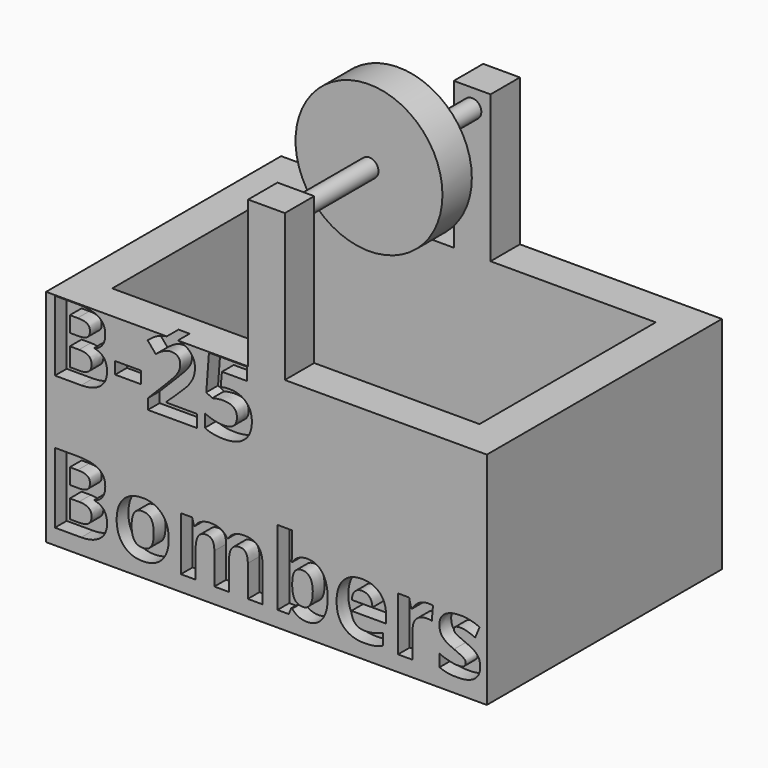
from build123d import *

# Parameters (mm, degrees)
F0_W          = 152.4
F0_H          = 76.2
F1_DEPTH      = 101.6
F2_W          = 127
F2_H          = 76.2
F3_DEPTH      = 63.5
F4_W          = 76.2
F4_H          = 25.4
F5_DEPTH      = 12.7
F6_W          = 12.7
F6_H          = 12.7
F7_DEPTH      = 50.8
F8_W          = 12.7
F8_H          = 12.7
F9_DEPTH      = 50.8
F10_R         = 3.175
F11_DEPTH     = 101.6
F13_R         = 25.4
F14_DEPTH     = 6.35
F15_R         = 6.35
F16_DEPTH     = 76.2
F17_TEXT_SIZE = 34.039085564
F18_DEPTH     = 5.08


# Not quite as in the source:
# - Text() gives the source's letters only with a copy of the font that has no kerning and outlines rounded to 1/6400 em; it was checked with that copy


with BuildPart() as f1:
    # F0 (on Front) → F1 (new body)
    with BuildSketch(Plane.XZ):
        with Locations((76.2, 38.1)):
            Rectangle(F0_W, F0_H)
    extrude(amount=-F1_DEPTH)

    # F2 (on face) → F3 (cut)
    with BuildSketch(Plane.XY.offset(76.2)):
        with Locations((76.2, 50.8)):
            Rectangle(F2_W, F2_H)
    extrude(amount=-F3_DEPTH, mode=Mode.SUBTRACT)

    # F4 (on face) → F5 (cut)
    with BuildSketch(Plane.XY.offset(12.7)):
        with Locations((76.2, 50.8)):
            Rectangle(F4_W, F4_H)
    extrude(amount=-F5_DEPTH, mode=Mode.SUBTRACT)

    # F6 (on face) → F7 (join)
    with BuildSketch(Plane.XY.offset(76.2)):
        with Locations((76.2, 95.25)):
            Rectangle(F6_W, F6_H)
    extrude(amount=F7_DEPTH)

    # F8 (on face) → F9 (join)
    with BuildSketch(Plane.XY.offset(76.2)):
        with Locations((76.2, 6.35)):
            Rectangle(F8_W, F8_H)
    extrude(amount=F9_DEPTH)

    # F10 (on face) → F11 (join)
    with BuildSketch(Plane.XZ):
        with Locations((76.2, 120.65)):
            Circle(F10_R)
    extrude(amount=-F11_DEPTH)

    # F13 (on offset) → F14 (join, symmetric)
    with BuildSketch(Plane.XZ.offset(-50.8)):
        with Locations((76.0903634732, 120.653526699)):
            Circle(F13_R)
    extrude(amount=F14_DEPTH, both=True)

    # F15 (on face) → F16 (join)
    with BuildSketch(Plane.XZ.offset(-88.9)):
        with Locations((121.0611678508, 19.1442768503)):
            Circle(F15_R)
    extrude(amount=F16_DEPTH)

    # F17 (on face) → F18 (cut)
    with BuildSketch(Plane.XZ):
        with Locations((0, 51.6918583939)):
            Text('B-25', F17_TEXT_SIZE, font='Open Sans', font_style=FontStyle.BOLD, text_align=(TextAlign.LEFT, TextAlign.BOTTOM))
        with Locations((0, 5.3987020269)):
            Text('Bombers', F17_TEXT_SIZE, font='Open Sans', font_style=FontStyle.BOLD, text_align=(TextAlign.LEFT, TextAlign.BOTTOM))
    extrude(amount=-F18_DEPTH, mode=Mode.SUBTRACT)


solid = f1.part
